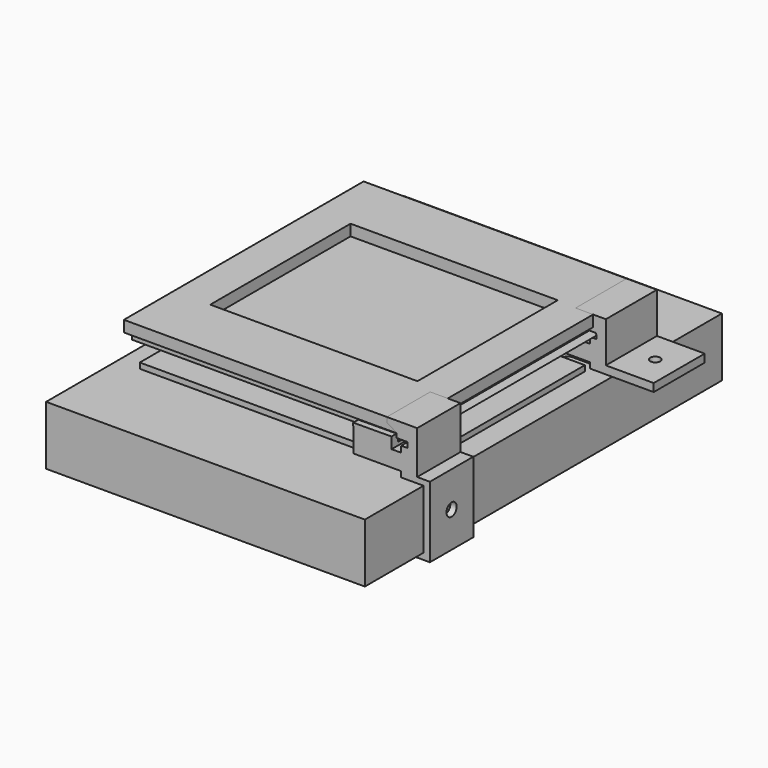
from build123d import *

# Parameters (mm, degrees)
F0_W           = 100
F0_H           = 140
F1_DEPTH       = 18.5
F3_DEPTH       = 1.75
F4_W           = 65
F4_H           = 55
F5_DEPTH       = 10
F6_W           = 88
F6_H           = 94
F6_W_2         = 86
F6_H_2         = 84
F6_W_3         = 65
F6_H_3         = 55
F6_H_4         = 3
F7_DEPTH       = 3.5
F8_DEPTH       = 2.5
F9_W           = 1
F9_H           = 1.25
F10_DEPTH      = 42
F10_DEPTH_BACK = 42
F12_DEPTH      = 47
F13_DEPTH      = 30
F15_DEPTH      = 12
F16_R          = 2
F17_DEPTH      = 3
F20_DEPTH      = 20
F21_R          = 1.55
F22_DEPTH      = 25


with BuildPart() as f1:
    # F0 (on Top) → F1 (new body)
    with BuildSketch(Plane.XY):
        Rectangle(F0_W, F0_H)
    extrude(amount=-F1_DEPTH)


with BuildPart() as f3:
    # F2 (on Top) → F3 (new body)
    with BuildSketch(Plane.XY):
        with BuildLine():
            Line((43, 42), (-43, 42))
            Line((-43, 42), (-43, 29))
            Line((-43, 29), (-36, 29))
            ThreePointArc((-36, 29), (-34, 27), (-36, 25))
            Line((-36, 25), (-43, 25))
            Line((-43, 25), (-43, -25))
            Line((-43, -25), (-36, -25))
            ThreePointArc((-36, -25), (-34, -27), (-36, -29))
            Line((-36, -29), (-43, -29))
            Line((-43, -29), (-43, -42))
            Line((-43, -42), (43, -42))
            Line((43, -42), (43, -29))
            Line((43, -29), (36, -29))
            ThreePointArc((36, -29), (34, -27), (36, -25))
            Line((36, -25), (43, -25))
            Line((43, -25), (43, 25))
            Line((43, 25), (36, 25))
            ThreePointArc((36, 25), (34, 27), (36, 29))
            Line((36, 29), (43, 29))
            Line((43, 29), (43, 42))
        make_face()
    extrude(amount=F3_DEPTH)


with BuildPart() as f5:
    # F4 (on face) → F5 (new body)
    with BuildSketch(Plane.XY.offset(1.75)):
        Rectangle(F4_W, F4_H)
    extrude(amount=F5_DEPTH)


with BuildPart() as f7:
    # F6 (on face) → F7 (new body)
    with BuildSketch(Plane.XY.offset(11.75)):
        Rectangle(F6_W, F6_H)
        Polygon((-43, 42), (-43, 45), (43, 45), (43, 42), (43, -42), (43, -44), (43, -45), (-43, -45), (-43, -44), (-43, -42), align=None, mode=Mode.SUBTRACT)
        Rectangle(F6_W_2, F6_H_2)
        Rectangle(F6_W_3, F6_H_3, mode=Mode.SUBTRACT)
        with Locations((0, 43.5)):
            Rectangle(F6_W_2, F6_H_4)
        Polygon((43, -42), (-43, -42), (-43, -44), (-43, -45), (43, -45), (43, -44), align=None)
    extrude(amount=F7_DEPTH)

    # F6 (on face) → F8 (join)
    with BuildSketch(Plane.XY.offset(11.75)):
        with Locations((0, 43.5)):
            Rectangle(F6_W_2, F6_H_4)
        Polygon((43, -42), (-43, -42), (-43, -44), (-43, -45), (43, -45), (43, -44), align=None)
    extrude(amount=-F8_DEPTH)

    # F9 (on Front) → F10 (join, two sides)
    with BuildSketch(Plane.XZ) as f10_sk:
        with Locations((42.5, 9.125)):
            Rectangle(F9_W, F9_H)
        Polygon((43, 9.75), (43, 8.5), (45, 9.75), align=None)
    extrude(amount=F10_DEPTH)
    extrude(f10_sk.sketch, amount=-F10_DEPTH_BACK)


with BuildPart() as f12:
    # F11 (on Front) → F12 (new body)
    with BuildSketch(Plane.XZ):
        Polygon((27.9699712028, 6.7499098263), (28, 1.75), (43, 1.75), (43, 0), (48, 0), (50, 0), (52, 0), (52, 1.75), (48, 1.75), (48, 13.75), (48, 15.25), (38.5, 15.25), (38.5, 13.75), (41.5, 11.875), (41.5, 10.4472711682), (44.9731051922, 10.4472711682), (45, 8.7854899466), (43, 8.7531212961), (43, 6.8401781918), align=None)
        Polygon((52, 0), (50, 0), (50, -18.5), (35.7036739588, -18.5), (35.7036739588, -20.5), (52, -20.5), align=None)
    extrude(amount=F12_DEPTH)

    # F11 (on Front) → F13 (cut)
    with BuildSketch(Plane.XZ):
        Polygon((27.9699712028, 6.7499098263), (28, 1.75), (43, 1.75), (43, 0), (48, 0), (50, 0), (52, 0), (52, 1.75), (48, 1.75), (48, 13.75), (48, 15.25), (38.5, 15.25), (38.5, 13.75), (41.5, 11.875), (41.5, 10.4472711682), (44.9731051922, 10.4472711682), (45, 8.7854899466), (43, 8.7531212961), (43, 6.8401781918), align=None)
        Polygon((52, 0), (50, 0), (50, -18.5), (35.7036739588, -18.5), (35.7036739588, -20.5), (52, -20.5), align=None)
    extrude(amount=F13_DEPTH, mode=Mode.SUBTRACT)

    # F14 (on face) → F15 (join)
    with BuildSketch(Plane(origin=(28.0094999534, 0, 0.1682213529), x_dir=(0, -1, 0), z_dir=(-0.9999819653, 0, -0.0060057594))):
        Polygon((39.5, 5.9370710514), (47, 5.9370710514), (47, 7.0816674463), (47, 10.0810629427), (44.5, 10.0810629427), (44.5, 7.5816674463), (42, 7.5816674463), (42, 9.5810629427), (42, 10.0810629427), (39.5, 10.0810629427), (39.5, 9.5810629427), align=None)
    extrude(amount=-F15_DEPTH)

    # F16 (on face) → F17 (cut)
    with BuildSketch(Plane.YZ.offset(52)):
        with Locations((-38.5, -9.375)):
            Circle(F16_R)
    extrude(amount=-F17_DEPTH, mode=Mode.SUBTRACT)


with BuildPart() as f20:
    # F19 (on offset) → F20 (new body)
    with BuildSketch(Plane(origin=(0, 27, 0), x_dir=(-1, 0, 0), z_dir=(0, 1, 0))):
        Polygon((-43, 1.75), (-28, 1.75), (-27.9699712028, 6.7499098263), (-43, 6.8401781918), (-43, 8.7531212961), (-45, 8.7854899466), (-44.9731051922, 10.4472711682), (-41.5, 10.4472711682), (-41.5, 11.875), (-38.5, 13.75), (-38.5, 15.25), (-48, 15.25), (-48, 2.5), (-63, 2.5), (-63, 0), (-43, 0), align=None)
    extrude(amount=F20_DEPTH)

    # F21 (on face) → F22 (cut)
    with BuildSketch(Plane.XY.offset(2.5)):
        with Locations((55.5, 37)):
            Circle(F21_R)
    extrude(amount=-F22_DEPTH, mode=Mode.SUBTRACT)


solid = Compound([f1.part, f3.part, f5.part, f7.part, f12.part, f20.part])
